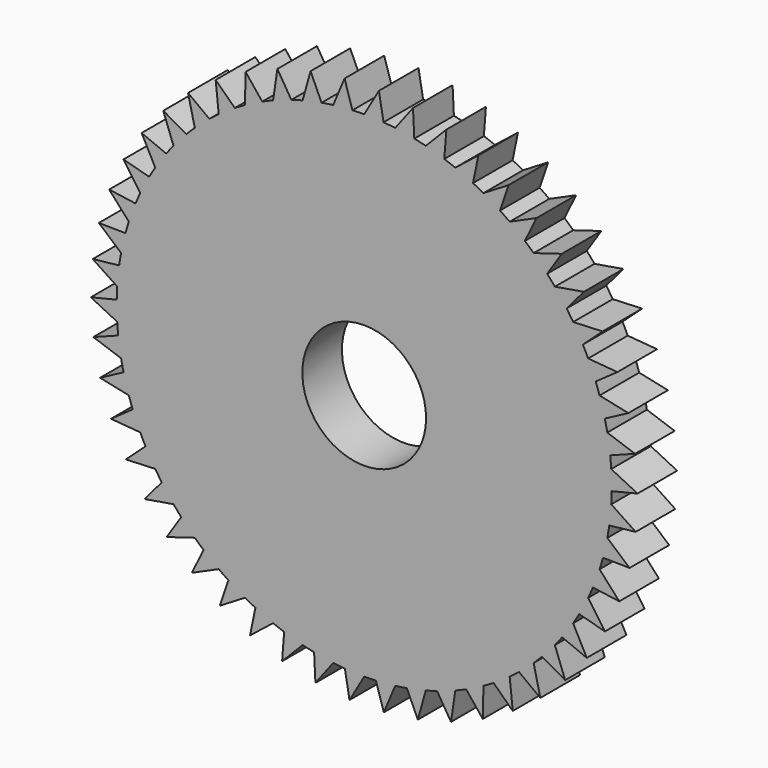
from build123d import *

# Parameters (mm, degrees)
F1_DEPTH        = 10
F2_DEPTH        = 10
F2_COPIES_COUNT = 50


# Not quite as in the source:
# - a pattern or mirror of a feature is missing from the dataset's text; its kind, count and spacing are read off the source's solid


with BuildPart() as f1:
    # F0 (on Front) → F1 (new body)
    with BuildSketch(Plane.XZ):
        with BuildLine():
            ThreePointArc((0, 50), (-35.3553390593, -35.3553390593), (50, 0))
            ThreePointArc((50, 0), (36.7094642634, 33.947241913), (3.9033906601, 49.8474025537))
            ThreePointArc((3.9033906601, 49.8474025537), (1.9531861551, 49.9618360736), (0, 50))
        make_face()
        with BuildLine():
            ThreePointArc((12.5, 0), (-8.8388347648, -8.8388347648), (0, 12.5))
            ThreePointArc((0, 12.5), (8.8388347648, 8.8388347648), (12.5, 0))
        make_face(mode=Mode.SUBTRACT)
    extrude(amount=F1_DEPTH)

    # F0 (on Front) → F2 (join)
    with BuildSketch(Plane.XZ):
        with BuildLine():
            ThreePointArc((0, 50), (1.9531861551, 49.9618360736), (3.9033906601, 49.8474025537))
            Line((3.9033906601, 49.8474025537), (2.9695587307, 55.1434265976))
            Line((2.9695587307, 55.1434265976), (0, 50))
        make_face()
    f2 = extrude(amount=F2_DEPTH)

    # F2_copies: F2 ×50 about axis
    f2_copies_axis = Axis((0, 0, 0), (0, 1, 0))
    for i in range(1, F2_COPIES_COUNT):
        add(f2.rotate(f2_copies_axis, i * 360 / F2_COPIES_COUNT))


solid = f1.part
